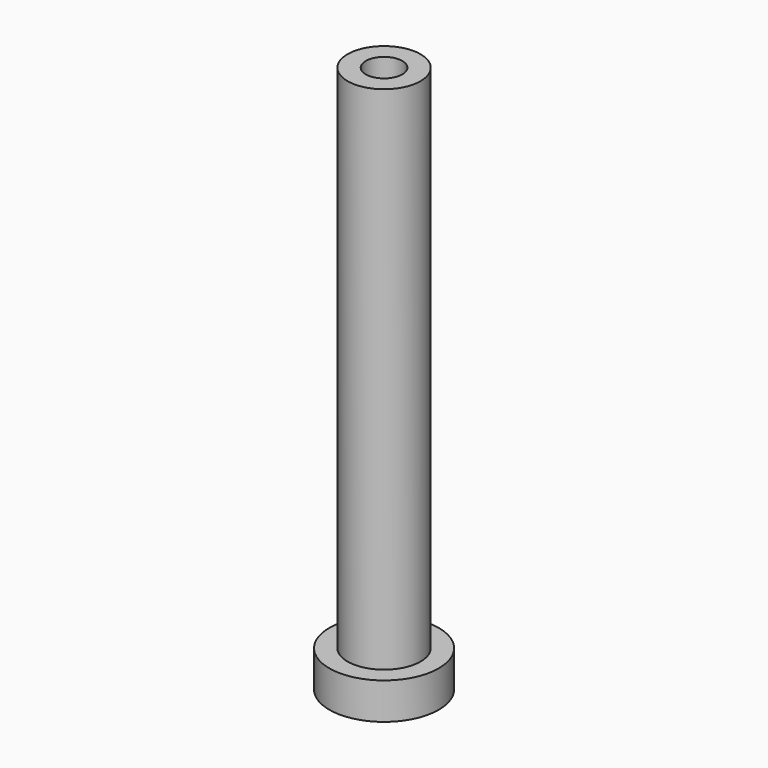
from build123d import *

# Parameters (mm, degrees)
F0_R     = 5
F1_DEPTH = 70
F2_R     = 7.5
F2_R_2   = 5
F3_DEPTH = 5
F4_R     = 2.5
F5_DEPTH = 25


with BuildPart() as f1:
    # F0 (on Top) → F1 (new body)
    with BuildSketch(Plane.XY):
        Circle(F0_R)
    extrude(amount=F1_DEPTH)

    # F2 (on face) → F3 (join)
    with BuildSketch(Plane(origin=(0, 0, 0), x_dir=(1, 0, 0), z_dir=(0, 0, -1))):
        Circle(F2_R)
        Circle(F2_R_2, mode=Mode.SUBTRACT)
        Circle(F2_R_2)
    extrude(amount=F3_DEPTH)

    # F4 (on face) → F5 (cut)
    with BuildSketch(Plane.XY.offset(70)):
        Circle(F4_R)
    extrude(amount=-F5_DEPTH, mode=Mode.SUBTRACT)


solid = f1.part
